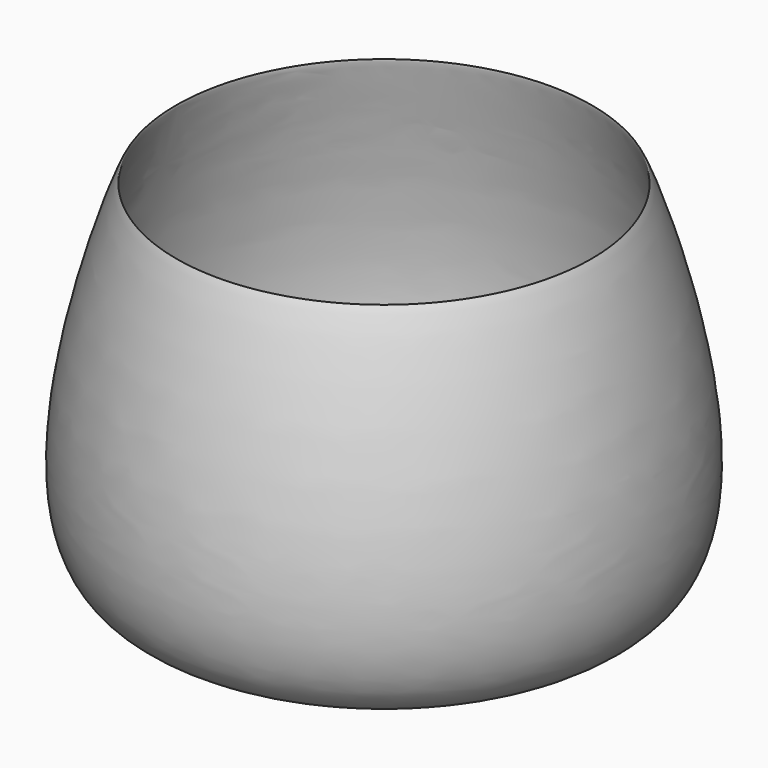
from build123d import *


# Not quite as in the source:
# - the program builds the solid bodies; features that only make, move or delete a surface that nothing else refers to are left out


with BuildPart() as f4:
    # F3 (on Front) → F4 (revolve)
    with BuildSketch(Plane.XZ):
        with BuildLine():
            add(Edge.make_bspline(
                [(-3.8956634235, 92.9549857974), (-4.0261143348, 92.7354124093), (-57.965781416, 72.9175607424), (-17.9283269619, 182.3816834796), (-52.907871745, 75.8425552097), (-3.7717697141, 93.1635221829), (-3.8956634235, 92.9549857974)],
                knots=[0, 0, 0, 0, 0.2251095736, 0.5076095041, 0.7862057091, 1, 1, 1, 1], degree=3))
        make_face()
    revolve(axis=Axis((0, 0, 104.1134409606), (0, 0, -1)))


solid = f4.part
